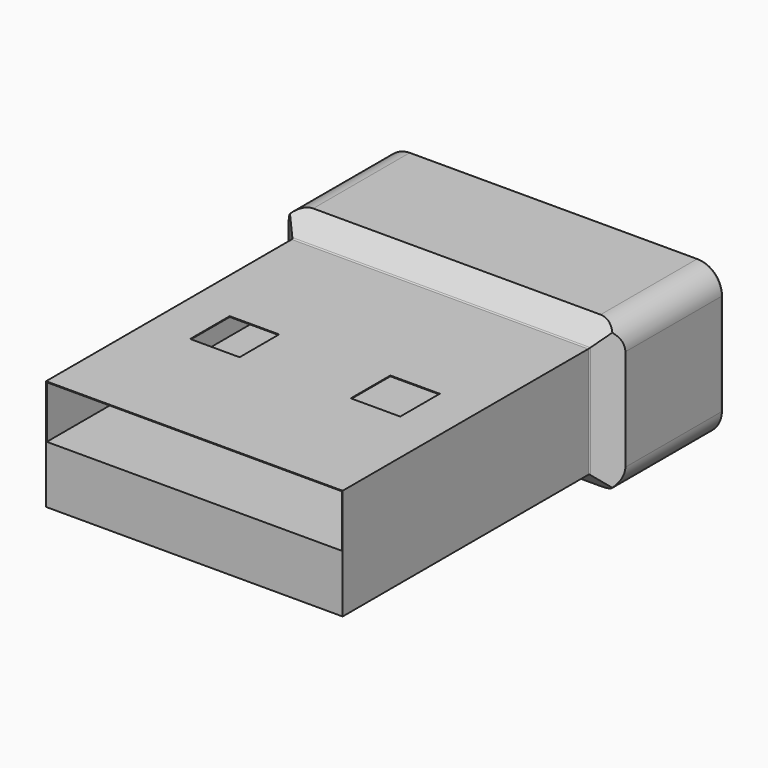
from build123d import *

# Parameters (mm, degrees)
F0_W         = 12
F0_H         = 4.48
F1_DEPTH     = 5.75
F0_W_2       = 11.94
F0_H_2       = 2.3
F2_DEPTH     = 5.75
F3_W         = 13.63
F3_H         = 6.11
F3_W_2       = 12
F3_H_2       = 4.48
F3_W_3       = 11.94
F3_H_3       = 2.12
F4_DEPTH     = 6.73
F5_T4_DEPTH  = 22.7851914372
F5_T9_DEPTH  = 22.7851914372
F5_T14_DEPTH = 22.7851914372
F5_T19_DEPTH = 15.2651914372
F5_T24_DEPTH = 15.2651914372
F5_T29_DEPTH = 15.2651914372
F5_T34_DEPTH = 22.7851914372
F5_T39_DEPTH = 22.7851914372
F5_T44_DEPTH = 22.7851914372
F5_T49_DEPTH = 15.2651914372
F5_T54_DEPTH = 15.2651914372
F5_T59_DEPTH = 15.2651914372
F6_R         = 0.1
F7_R         = 1
F8_R         = 0.1
F9_W         = 2
F9_H         = 2
F10_DEPTH    = 2.15
F11_W        = 0.001
F11_H        = 12.4235786438
F12_DEPTH    = 0.3


# Not quite as in the source:
# - a fillet or chamfer that OpenCascade refuses, or shapes differently, is made with other operations: its cross-section is extruded or revolved along the edge and cut away or added


with BuildPart() as f1:
    # F0 (on Front) → F1 (new body, symmetric)
    with BuildSketch(Plane.XZ):
        Rectangle(F0_W, F0_H)
        Polygon((5.97, -2.21), (-5.97, -2.21), (-5.97, 0.09), (-5.97, 2.21), (5.97, 2.21), (5.97, 0.09), align=None, mode=Mode.SUBTRACT)
    extrude(amount=F1_DEPTH, both=True)

    # F0 (on Front) → F2 (join, symmetric)
    with BuildSketch(Plane.XZ):
        with Locations((0, -1.06)):
            Rectangle(F0_W_2, F0_H_2)
    extrude(amount=F2_DEPTH, both=True)

    # F3 (on face) → F4 (join)
    with BuildSketch(Plane(origin=(0, 5.75, 0), x_dir=(-1, 0, 0), z_dir=(0, 1, 0))):
        Rectangle(F3_W, F3_H)
        Rectangle(F3_W_2, F3_H_2, mode=Mode.SUBTRACT)
        Rectangle(F3_W_2, F3_H_2)
        with Locations((0, 1.15)):
            Rectangle(F3_W_3, F3_H_3, mode=Mode.SUBTRACT)
        with Locations((0, 1.15)):
            Rectangle(F3_W_3, F3_H_3)
    extrude(amount=F4_DEPTH)

    # F5: chamfer of 1.78 on 4 edges, made by hand


with BuildPart() as f5_tool2:
    # F5_s3 → F5_t4 (new body)
    with BuildSketch(Plane.YZ.offset(-11.3925957186)):
        Polygon((5.75, 1.275), (7.53, 3.055), (5.75, 3.055), align=None)
    extrude(amount=F5_T4_DEPTH)

    split(bisect_by=Plane.YZ.offset(-6), keep=Keep.BOTTOM)


with BuildPart() as f1_1:
    add(f1.part)

    # F5_t1: cut F5_tool2
    add(f5_tool2.part, mode=Mode.SUBTRACT)


with BuildPart() as f5_tool7:
    # F5_s8 → F5_t9 (new body)
    with BuildSketch(Plane.YZ.offset(-11.3925957186)):
        Polygon((5.75, 1.275), (7.53, 3.055), (5.75, 3.055), align=None)
    extrude(amount=F5_T9_DEPTH)

    split(bisect_by=Plane.XY.offset(2.24), keep=Keep.TOP)


with BuildPart() as f1_2:
    add(f1_1.part)

    # F5_t6: cut F5_tool7
    add(f5_tool7.part, mode=Mode.SUBTRACT)


with BuildPart() as f5_tool12:
    # F5_s13 → F5_t14 (new body)
    with BuildSketch(Plane.YZ.offset(-11.3925957186)):
        Polygon((5.75, 1.275), (7.53, 3.055), (5.75, 3.055), align=None)
    extrude(amount=F5_T14_DEPTH)

    split(bisect_by=Plane.YZ.offset(6), keep=Keep.TOP)


with BuildPart() as f1_3:
    add(f1_2.part)

    # F5_t11: cut F5_tool12
    add(f5_tool12.part, mode=Mode.SUBTRACT)


with BuildPart() as f5_tool17:
    # F5_s18 → F5_t19 (new body)
    with BuildSketch(Plane.XY.offset(7.6325957186)):
        Polygon((6.815, 7.53), (5.035, 5.75), (6.815, 5.75), align=None)
    extrude(amount=-F5_T19_DEPTH)

    split(bisect_by=Plane.YZ.offset(6), keep=Keep.TOP)


with BuildPart() as f1_4:
    add(f1_3.part)

    # F5_t16: cut F5_tool17
    add(f5_tool17.part, mode=Mode.SUBTRACT)


with BuildPart() as f5_tool22:
    # F5_s23 → F5_t24 (new body)
    with BuildSketch(Plane.XY.offset(7.6325957186)):
        Polygon((6.815, 7.53), (5.035, 5.75), (6.815, 5.75), align=None)
    extrude(amount=-F5_T24_DEPTH)

    split(bisect_by=Plane.XY.offset(2.24), keep=Keep.TOP)


with BuildPart() as f1_5:
    add(f1_4.part)

    # F5_t21: cut F5_tool22
    add(f5_tool22.part, mode=Mode.SUBTRACT)


with BuildPart() as f5_tool27:
    # F5_s28 → F5_t29 (new body)
    with BuildSketch(Plane.XY.offset(7.6325957186)):
        Polygon((6.815, 7.53), (5.035, 5.75), (6.815, 5.75), align=None)
    extrude(amount=-F5_T29_DEPTH)

    split(bisect_by=Plane.XY.offset(-2.24), keep=Keep.BOTTOM)


with BuildPart() as f1_6:
    add(f1_5.part)

    # F5_t26: cut F5_tool27
    add(f5_tool27.part, mode=Mode.SUBTRACT)


with BuildPart() as f5_tool32:
    # F5_s33 → F5_t34 (new body)
    with BuildSketch(Plane.YZ.offset(11.3925957186)):
        Polygon((7.53, -3.055), (5.75, -1.275), (5.75, -3.055), align=None)
    extrude(amount=-F5_T34_DEPTH)

    split(bisect_by=Plane.XY.offset(-2.24), keep=Keep.BOTTOM)


with BuildPart() as f1_7:
    add(f1_6.part)

    # F5_t31: cut F5_tool32
    add(f5_tool32.part, mode=Mode.SUBTRACT)


with BuildPart() as f5_tool37:
    # F5_s38 → F5_t39 (new body)
    with BuildSketch(Plane.YZ.offset(11.3925957186)):
        Polygon((7.53, -3.055), (5.75, -1.275), (5.75, -3.055), align=None)
    extrude(amount=-F5_T39_DEPTH)

    split(bisect_by=Plane.YZ.offset(6), keep=Keep.TOP)


with BuildPart() as f1_8:
    add(f1_7.part)

    # F5_t36: cut F5_tool37
    add(f5_tool37.part, mode=Mode.SUBTRACT)


with BuildPart() as f5_tool42:
    # F5_s43 → F5_t44 (new body)
    with BuildSketch(Plane.YZ.offset(11.3925957186)):
        Polygon((7.53, -3.055), (5.75, -1.275), (5.75, -3.055), align=None)
    extrude(amount=-F5_T44_DEPTH)

    split(bisect_by=Plane.YZ.offset(-6), keep=Keep.BOTTOM)


with BuildPart() as f1_9:
    add(f1_8.part)

    # F5_t41: cut F5_tool42
    add(f5_tool42.part, mode=Mode.SUBTRACT)


with BuildPart() as f5_tool47:
    # F5_s48 → F5_t49 (new body)
    with BuildSketch(Plane.XY.offset(-7.6325957186)):
        Polygon((-6.815, 7.53), (-5.035, 5.75), (-6.815, 5.75), align=None)
    extrude(amount=F5_T49_DEPTH)

    split(bisect_by=Plane.YZ.offset(-6), keep=Keep.BOTTOM)


with BuildPart() as f1_10:
    add(f1_9.part)

    # F5_t46: cut F5_tool47
    add(f5_tool47.part, mode=Mode.SUBTRACT)


with BuildPart() as f5_tool52:
    # F5_s53 → F5_t54 (new body)
    with BuildSketch(Plane.XY.offset(-7.6325957186)):
        Polygon((-6.815, 7.53), (-5.035, 5.75), (-6.815, 5.75), align=None)
    extrude(amount=F5_T54_DEPTH)

    split(bisect_by=Plane.XY.offset(-2.24), keep=Keep.BOTTOM)


with BuildPart() as f1_11:
    add(f1_10.part)

    # F5_t51: cut F5_tool52
    add(f5_tool52.part, mode=Mode.SUBTRACT)


with BuildPart() as f5_tool57:
    # F5_s58 → F5_t59 (new body)
    with BuildSketch(Plane.XY.offset(-7.6325957186)):
        Polygon((-6.815, 7.53), (-5.035, 5.75), (-6.815, 5.75), align=None)
    extrude(amount=F5_T59_DEPTH)

    split(bisect_by=Plane.XY.offset(2.24), keep=Keep.TOP)


with BuildPart() as f1_12:
    add(f1_11.part)

    # F5_t56: cut F5_tool57
    add(f5_tool57.part, mode=Mode.SUBTRACT)

    # F6
    f6_edges = [f1_12.edges().sort_by_distance(p)[0] for p in [
        (0, 6.715, 2.24),
        (6, 6.715, 0),
        (-6, 6.715, 0),
        (0, 6.715, -2.24),
    ]]
    fillet(f6_edges, radius=F6_R)

    # F7
    f7_edges = [f1_12.edges().sort_by_distance(p)[0] for p in [
        (-6.815, 10.005, -3.055),
        (-6.815, 10.005, 3.055),
        (6.815, 10.005, -3.055),
        (6.815, 10.005, 3.055),
    ]]
    fillet(f7_edges, radius=F7_R)

    # F8
    f8_edges = [f1_12.edges().sort_by_distance(p)[0] for p in [
        (0, 12.48, 3.055),
        (-6.522107, 12.48, 2.762107),
        (6.522107, 12.48, 2.762107),
        (-6.522107, 12.48, -2.762107),
        (-6.815, 12.48, 0),
        (0, 12.48, -3.055),
        (6.522107, 12.48, -2.762107),
        (6.815, 12.48, 0),
    ]]
    fillet(f8_edges, radius=F8_R)

    # F9 (on face) → F10 (cut, through all)
    with BuildSketch(Plane.XY.offset(2.24)):
        with Locations((-3.25, 0.35)):
            Rectangle(F9_W, F9_H)
        with Locations((3.25, 0.35)):
            Rectangle(F9_W, F9_H)
    extrude(amount=-F10_DEPTH, mode=Mode.SUBTRACT)

    # F11 (on face) → F12 (cut)
    with BuildSketch(Plane(origin=(0, 0, -2.24), x_dir=(1, 0, 0), z_dir=(0, 0, -1))):
        with Locations((0.0005, -0.4617893219)):
            Rectangle(F11_W, F11_H)
        with Locations((-0.0005, -0.4617893219)):
            Rectangle(F11_W, F11_H)
    extrude(amount=-F12_DEPTH, mode=Mode.SUBTRACT)


solid = f1_12.part
